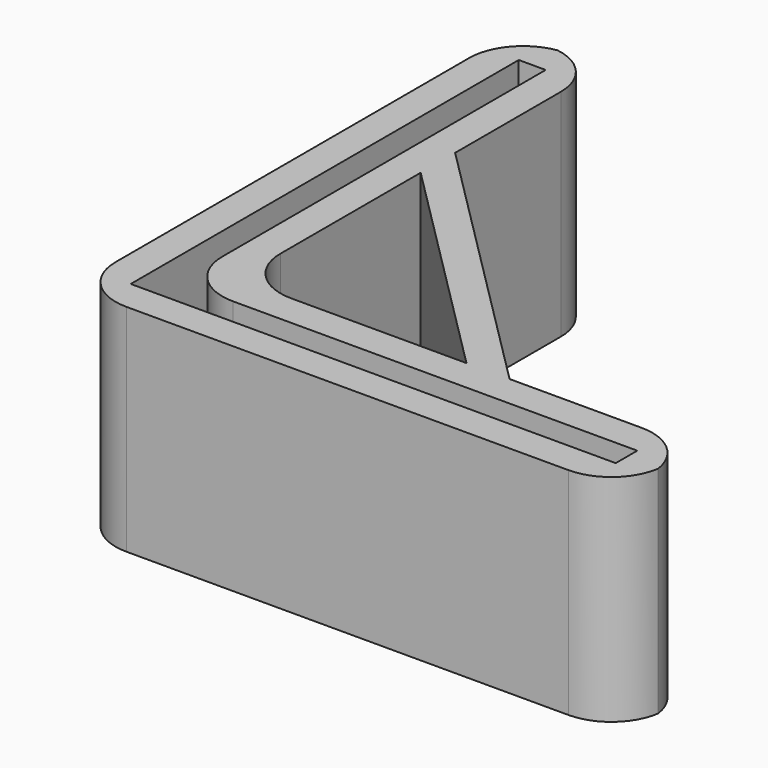
from build123d import *

# Parameters (mm, degrees)
F1_DEPTH    = 20
F2_DEPTH    = 6
F3_T1_DEPTH = 20
F3_T3_DEPTH = 45
F4_R        = 5


# Not quite as in the source:
# - a fillet or chamfer that OpenCascade refuses, or shapes differently, is made with other operations: its cross-section is extruded or revolved along the edge and cut away or added


with BuildPart() as f1:
    # F0 (on Top) → F1 (new body)
    with BuildSketch(Plane.XY):
        Polygon((5.5, 30.75), (5.5, 48), (-3, 48), (-3, -3), (48, -3), (48, 5.5), (30.75, 5.5), (26.75, 5.5), (5.5, 5.5), (5.5, 26.75), align=None)
        Polygon((0, 0), (0, 45), (2.5, 45), (2.5, 2.5), (45, 2.5), (45, 0), align=None, mode=Mode.SUBTRACT)
        Polygon((30.75, 5.5), (5.5, 30.75), (5.5, 26.75), (26.75, 5.5), align=None)
    extrude(amount=F1_DEPTH)

    # F0 (on Top) → F2 (join)
    with BuildSketch(Plane.XY):
        Polygon((2.5, 45), (0, 45), (0, 0), (45, 0), (45, 2.5), (2.5, 2.5), align=None)
    extrude(amount=F2_DEPTH)

    # F3: fillet of radius 5 on 6 edges, made by hand

    # F3_s2 → F3_t1 (join)
    with BuildSketch(Plane.XY):
        with BuildLine():
            ThreePointArc((10.5, 5.5), (6.9644660941, 6.9644660941), (5.5, 10.5))
            Line((5.5, 10.5), (5.5, 5.5))
            Line((5.5, 5.5), (10.5, 5.5))
        make_face()
    extrude(amount=F3_T1_DEPTH)

    # F3_s4 → F3_t3 (cut)
    with BuildSketch(Plane.XY.offset(-12.5)):
        with BuildLine():
            ThreePointArc((43, 5.5), (46.5355339059, 4.0355339059), (48, 0.5))
            Line((48, 0.5), (48, 5.5))
            Line((48, 5.5), (43, 5.5))
        make_face()
        with BuildLine():
            ThreePointArc((43, -3), (46.5355339059, -1.5355339059), (48, 2))
            Line((48, 2), (48, -3))
            Line((48, -3), (43, -3))
        make_face()
        with BuildLine():
            ThreePointArc((5.5, 43), (4.0355339059, 46.5355339059), (0.5, 48))
            Line((0.5, 48), (5.5, 48))
            Line((5.5, 48), (5.5, 43))
        make_face()
        with BuildLine():
            ThreePointArc((2, 48), (-1.5355339059, 46.5355339059), (-3, 43))
            Line((-3, 43), (-3, 48))
            Line((-3, 48), (2, 48))
        make_face()
        with BuildLine():
            ThreePointArc((-3, 2), (-1.5355339059, -1.5355339059), (2, -3))
            Line((2, -3), (-3, -3))
            Line((-3, -3), (-3, 2))
        make_face()
    extrude(amount=F3_T3_DEPTH, mode=Mode.SUBTRACT)

    # F4
    f4_edges = [f1.edges().sort_by_distance(p)[0] for p in [
        (2.5, 2.5, 13),
    ]]
    fillet(f4_edges, radius=F4_R)


solid = f1.part
